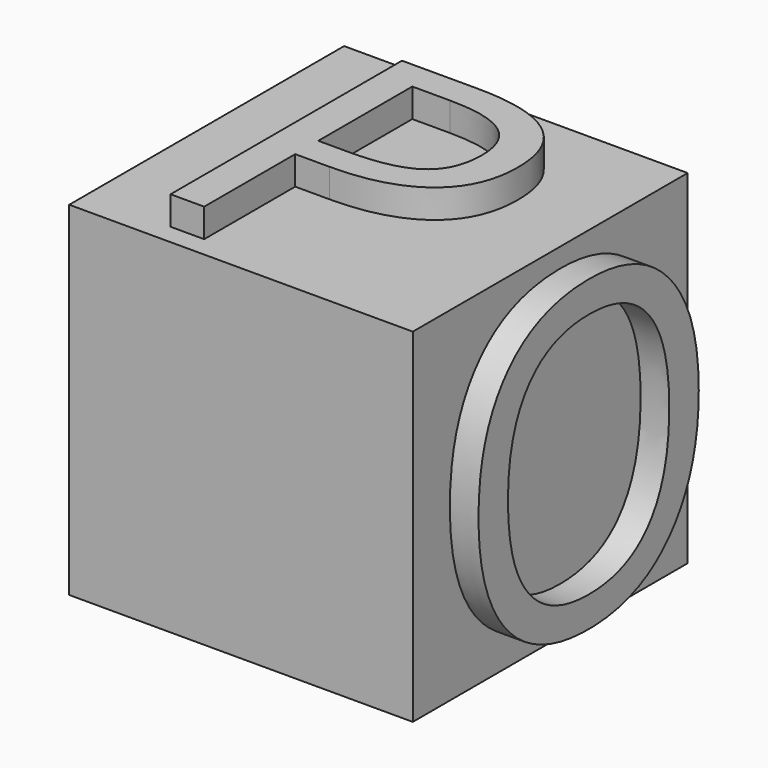
from build123d import *

# Parameters (mm, degrees)
F0_W         = 76.2
F0_H         = 76.2
F1_DEPTH     = 76.2
F3_T         = -2.54
F4_TEXT_SIZE = 89.8711532096
F5_DEPTH     = 6.35
F6_TEXT_SIZE = 92.9908180195
F7_DEPTH     = 6.35


# Not quite as in the source:
# - a feature names something its author has since deleted; it is built from what else it names
# - Text() gives the source's letters only with a copy of the font that has no kerning and outlines rounded to 1/6400 em; it was checked with that copy


with BuildPart() as f1:
    # F0 (on Front) → F1 (new body)
    with BuildSketch(Plane.XZ):
        with Locations((-2.7521848679, -6.6302279345)):
            Rectangle(F0_W, F0_H)
    extrude(amount=F1_DEPTH)

    # F3
    f3_openings = [f1.faces().sort_by_distance(p)[0] for p in [
        (-2.752185, 0, -6.630228),
    ]]
    offset(amount=F3_T, openings=f3_openings)

    # F4 (on face) → F5 (join)
    with BuildSketch(Plane.XY.offset(31.4697720655)):
        with Locations((-30.8024082333, -71.6943144798)):
            Text('P', F4_TEXT_SIZE, font='Open Sans', text_align=(TextAlign.LEFT, TextAlign.BOTTOM))
    extrude(amount=F5_DEPTH)

    # F6 (on face) → F7 (join)
    with BuildSketch(Plane.YZ.offset(35.3478151321)):
        with Locations((-71.606837213, -40.2469448745)):
            Text('O', F6_TEXT_SIZE, font='Open Sans', text_align=(TextAlign.LEFT, TextAlign.BOTTOM))
    extrude(amount=F7_DEPTH)


solid = f1.part
